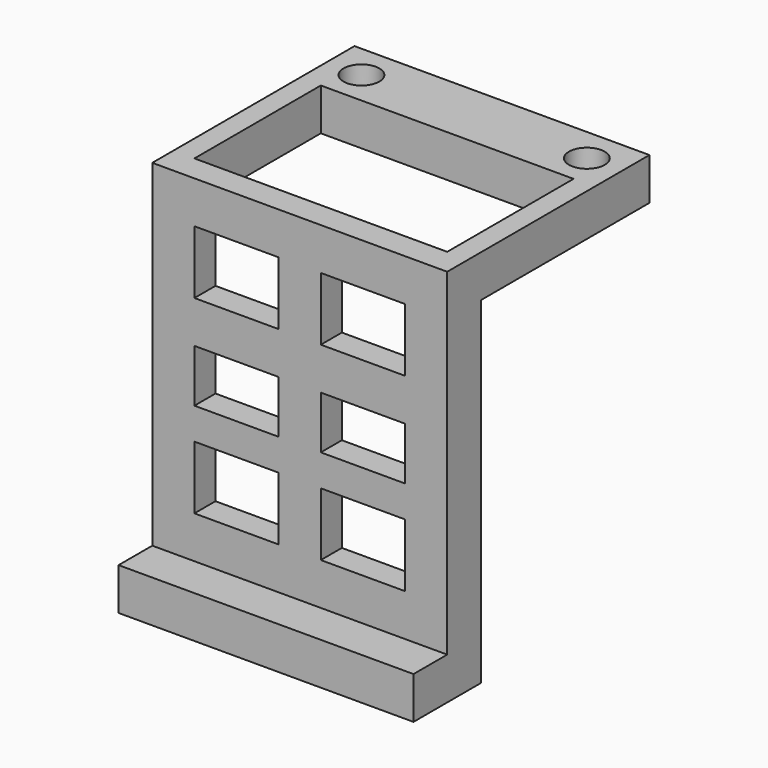
from build123d import *

# Parameters (mm, degrees)
F0_W     = 140
F0_H     = 140
F0_R     = 8.5
F0_W_2   = 120
F0_H_2   = 75
F1_DEPTH = 180
F2_W     = 20
F2_H     = 160
F2_W_2   = 100
F3_DEPTH = 140
F4_W     = 40
F4_H     = 30
F4_H_2   = 25
F5_DEPTH = 20


# Not quite as in the source:
# - a feature names something its author has since deleted; it is built from what else it names


with BuildPart() as f1:
    # F0 (on Top) → F1 (new body)
    with BuildSketch(Plane.XY):
        Rectangle(F0_W, F0_H)
        with Locations((-53.5, 53.5)):
            Circle(F0_R, mode=Mode.SUBTRACT)
        Rectangle(F0_W_2, F0_H_2, mode=Mode.SUBTRACT)
        with Locations((53.5, 53.5)):
            Circle(F0_R, mode=Mode.SUBTRACT)
    extrude(amount=F1_DEPTH)

    # F2 (on face) → F3 (cut)
    with BuildSketch(Plane.YZ.offset(70)):
        with Locations((-60, 100)):
            Rectangle(F2_W, F2_H)
        with Locations((20, 80)):
            Rectangle(F2_W_2, F2_H)
    extrude(amount=-F3_DEPTH, mode=Mode.SUBTRACT)

    # F4 (on face) → F5 (cut)
    with BuildSketch(Plane.XZ.offset(50)):
        with Locations((-30, 145)):
            Rectangle(F4_W, F4_H)
        with Locations((30, 145)):
            Rectangle(F4_W, F4_H)
        with Locations((30, 55)):
            Rectangle(F4_W, F4_H)
        with Locations((-30, 55)):
            Rectangle(F4_W, F4_H)
        with Locations((-30, 97.5)):
            Rectangle(F4_W, F4_H_2)
        with Locations((30, 97.5)):
            Rectangle(F4_W, F4_H_2)
    extrude(amount=-F5_DEPTH, mode=Mode.SUBTRACT)


solid = f1.part
